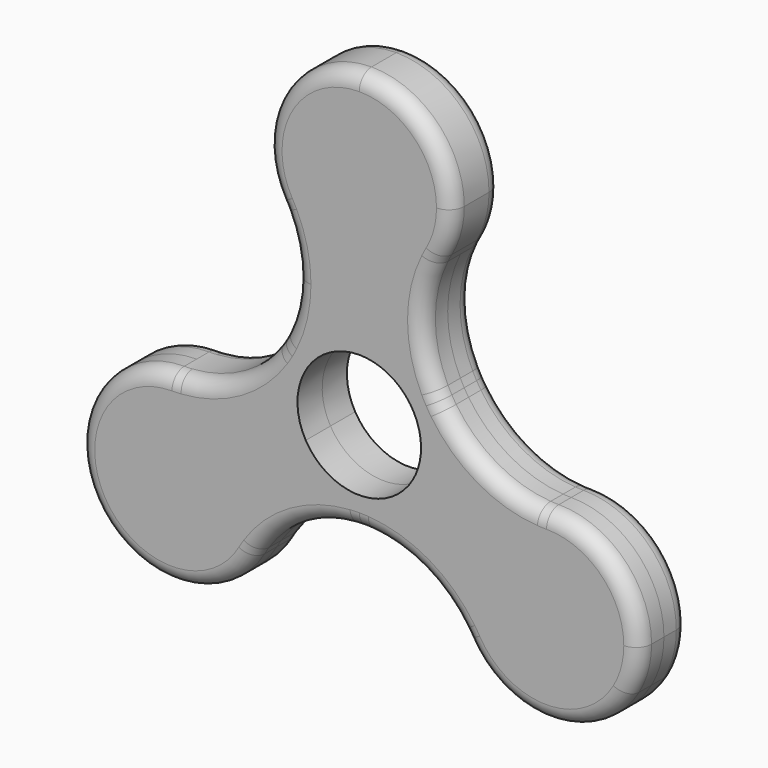
from build123d import *

# Parameters (mm, degrees)
F1_DEPTH = 2.54
F2_R     = 1.27


# Not quite as in the source:
# - a feature names something its author has since deleted; it is built from what else it names


with BuildPart() as f1:
    # F0 (on Front) → F1 (new body, symmetric)
    with BuildSketch(Plane.XZ):
        with BuildLine():
            ThreePointArc((7.62, 17.78), (5.3881536726, 23.1681536726), (0, 25.4))
            Line((0, 25.4), (0, 10.16))
            ThreePointArc((0, 10.16), (3.249178877, 10.887450644), (5.877985768, 12.9309090222))
            ThreePointArc((5.877985768, 12.9309090222), (6.260146038, 13.4354664712), (6.5991134209, 13.96999973))
            ThreePointArc((6.5991134209, 13.96999973), (7.360354756, 15.8077987257), (7.62, 17.78))
        make_face()
        with BuildLine():
            Line((0, 10.16), (0, 25.4))
            ThreePointArc((0, 25.4), (-6.5991135286, 21.5900000836), (-6.5991136733, 13.9700001671))
            ThreePointArc((-6.5991136733, 13.9700001671), (-6.2601461875, 13.4354666866), (-5.8779857805, 12.9309090373))
            ThreePointArc((-5.8779857805, 12.9309090373), (-3.2491788858, 10.8874506481), (0, 10.16))
        make_face()
        with BuildLine():
            Line((0, 7.62), (0, 10.16))
            ThreePointArc((0, 10.16), (-3.2491788858, 10.8874506481), (-5.8779857805, 12.9309090373))
            ThreePointArc((-5.8779857805, 12.9309090373), (-4.8002366489, 11.0368765758), (-4.4263073453, 8.89))
            ThreePointArc((-4.4263073453, 8.89), (-4.8002366648, 6.74312338), (-5.8779858402, 4.8490908903))
            ThreePointArc((-5.8779858402, 4.8490908903), (-3.2491789283, 6.8925493318), (0, 7.62))
        make_face()
        with BuildLine():
            ThreePointArc((5.877985768, 12.9309090222), (3.249178877, 10.887450644), (0, 10.16))
            Line((0, 10.16), (0, 7.62))
            ThreePointArc((0, 7.62), (3.2491789453, 6.8925493238), (5.8779858642, 4.8490908613))
            ThreePointArc((5.8779858642, 4.8490908613), (4.4263073453, 8.8899999245), (5.877985768, 12.9309090222))
        make_face()
        with BuildLine():
            ThreePointArc((-14.1374887376, -1.3749694884), (-11.0533983396, -2.6298538308), (-8.7988181024, -5.08))
            Line((-8.7988181024, -5.08), (-6.5991135768, -3.81))
            ThreePointArc((-6.5991135768, -3.81), (-7.5937122775, -0.6324032306), (-7.1384288571, 2.6659395065))
            ThreePointArc((-7.1384288571, 2.6659395065), (-9.9121195778, -0.6117054319), (-14.1374887376, -1.3749694884))
        make_face()
        with BuildLine():
            Line((-6.5991135768, -3.81), (-8.7988181024, -5.08))
            ThreePointArc((-8.7988181024, -5.08), (-8.037576883, -6.9177988763), (-7.7779316793, -8.89))
            ThreePointArc((-7.7779316793, -8.89), (-7.8992908924, -10.2445428561), (-8.2595028995, -11.5559397134))
            ThreePointArc((-8.2595028995, -11.5559397134), (-5.4858122449, -8.2782946509), (-1.2604430504, -7.5150304934))
            ThreePointArc((-1.2604430504, -7.5150304934), (-4.344533385, -6.2601461378), (-6.5991135768, -3.81))
        make_face()
        with BuildLine():
            ThreePointArc((-15.3979316793, -1.27), (-21.9970452561, -5.08), (-21.9970452561, -12.7))
            Line((-21.9970452561, -12.7), (-8.7988181024, -5.08))
            ThreePointArc((-8.7988181024, -5.08), (-11.0533983396, -2.6298538308), (-14.1374887376, -1.3749694884))
            ThreePointArc((-14.1374887376, -1.3749694884), (-14.7655285241, -1.2962877162), (-15.3979316793, -1.27))
        make_face()
        with BuildLine():
            Line((-8.7988181024, -5.08), (-21.9970452561, -12.7))
            ThreePointArc((-21.9970452561, -12.7), (-15.3979316818, -16.51), (-8.7988181049, -12.7000000043))
            ThreePointArc((-8.7988181049, -12.7000000043), (-8.5053823708, -12.1391789778), (-8.2595028995, -11.5559397134))
            ThreePointArc((-8.2595028995, -11.5559397134), (-7.8992908924, -10.2445428561), (-7.7779316793, -8.89))
            ThreePointArc((-7.7779316793, -8.89), (-8.037576883, -6.9177988763), (-8.7988181024, -5.08))
        make_face()
        with BuildLine():
            ThreePointArc((1.2604429732, -7.5150305063), (4.3445333529, -6.2601461601), (6.5991135768, -3.81))
            Line((6.5991135768, -3.81), (4.3994090512, -2.54))
            ThreePointArc((4.3994090512, -2.54), (0, -5.08), (-4.3994090512, -2.54))
            Line((-4.3994090512, -2.54), (-6.5991135768, -3.81))
            ThreePointArc((-6.5991135768, -3.81), (-4.344533385, -6.2601461378), (-1.2604430504, -7.5150304934))
            ThreePointArc((-1.2604430504, -7.5150304934), (-0.6324032184, -7.5937122785), (-1.66e-08, -7.62))
            ThreePointArc((-1.66e-08, -7.62), (0.6324031628, -7.5937122832), (1.2604429732, -7.5150305063))
        make_face()
        with BuildLine():
            Line((-6.5991135768, -3.81), (-4.3994090512, -2.54))
            ThreePointArc((-4.3994090512, -2.54), (-4.3994090512, 2.54), (0, 5.08))
            Line((0, 5.08), (0, 7.62))
            ThreePointArc((0, 7.62), (-3.2491789283, 6.8925493318), (-5.8779858402, 4.8490908903))
            ThreePointArc((-5.8779858402, 4.8490908903), (-6.2601461212, 4.3445334089), (-6.5991135101, 3.8100001156))
            ThreePointArc((-6.5991135101, 3.8100001156), (-6.8925493282, 3.249178936), (-7.1384288571, 2.6659395065))
            ThreePointArc((-7.1384288571, 2.6659395065), (-7.5937122775, -0.6324032306), (-6.5991135768, -3.81))
        make_face()
        with BuildLine():
            ThreePointArc((8.2595029011, -11.5559397177), (7.8042193924, -8.2575968818), (8.7988181024, -5.08))
            Line((8.7988181024, -5.08), (6.5991135768, -3.81))
            ThreePointArc((6.5991135768, -3.81), (4.3445333529, -6.2601461601), (1.2604429732, -7.5150305063))
            ThreePointArc((1.2604429732, -7.5150305063), (5.4858122129, -8.2782946325), (8.2595029011, -11.5559397177))
        make_face()
        with BuildLine():
            Line((6.5991135768, -3.81), (8.7988181024, -5.08))
            ThreePointArc((8.7988181024, -5.08), (11.0533983038, -2.6298538556), (14.1374886517, -1.3749695028))
            ThreePointArc((14.1374886517, -1.3749695028), (9.9121195513, -0.6117054166), (7.1384288662, 2.6659394822))
            ThreePointArc((7.1384288662, 2.6659394822), (7.4986408088, 1.3545427346), (7.62, 0))
            ThreePointArc((7.62, 0), (7.3603547963, -1.9722011237), (6.5991135768, -3.81))
        make_face()
        with BuildLine():
            Line((8.7988181024, -5.08), (21.9970452561, -12.7))
            ThreePointArc((21.9970452561, -12.7), (22.7582864756, -10.8622011237), (23.0179316793, -8.89))
            ThreePointArc((23.0179316793, -8.89), (20.7860853519, -3.5018463274), (15.3979316793, -1.27))
            ThreePointArc((15.3979316793, -1.27), (14.7655284807, -1.2962877198), (14.1374886517, -1.3749695028))
            ThreePointArc((14.1374886517, -1.3749695028), (11.0533983038, -2.6298538556), (8.7988181024, -5.08))
        make_face()
        with BuildLine():
            ThreePointArc((8.7988181117, -12.700000016), (15.3979316885, -16.51), (21.9970452561, -12.7))
            Line((21.9970452561, -12.7), (8.7988181024, -5.08))
            ThreePointArc((8.7988181024, -5.08), (7.8042193924, -8.2575968818), (8.2595029011, -11.5559397177))
            ThreePointArc((8.2595029011, -11.5559397177), (8.5053823746, -12.139178986), (8.7988181117, -12.700000016))
        make_face()
        with BuildLine():
            ThreePointArc((-14.7246582835, -1.2476675293), (-14.4325799527, -1.318266846), (-14.1374887376, -1.3749694884))
            ThreePointArc((-14.1374887376, -1.3749694884), (-9.9121195778, -0.6117054319), (-7.1384288571, 2.6659395065))
            ThreePointArc((-7.1384288571, 2.6659395065), (-7.0399891484, 2.9498473861), (-6.9550907617, 3.2380943709))
            ThreePointArc((-6.9550907617, 3.2380943709), (-10.3179316793, 0.0911818976), (-14.7246582835, -1.2476675293))
        make_face()
        with BuildLine():
            Line((4.3994090512, -2.54), (6.5991135768, -3.81))
            ThreePointArc((6.5991135768, -3.81), (7.3603547963, -1.9722011237), (7.62, 0))
            ThreePointArc((7.62, 0), (7.4986408088, 1.3545427346), (7.1384288662, 2.6659394822))
            ThreePointArc((7.1384288662, 2.6659394822), (6.8925492974, 3.2491790013), (6.5991134249, 3.8100002632))
            ThreePointArc((6.5991134249, 3.8100002632), (6.2601460834, 4.3445334634), (5.8779858642, 4.8490908613))
            ThreePointArc((5.8779858642, 4.8490908613), (3.2491789453, 6.8925493238), (0, 7.62))
            Line((0, 7.62), (0, 5.08))
            ThreePointArc((0, 5.08), (3.5921024484, 3.5921024484), (5.08, 0))
            ThreePointArc((5.08, 0), (4.9069031975, -1.3148007491), (4.3994090512, -2.54))
        make_face()
        with BuildLine():
            ThreePointArc((-1.2604430504, -7.5150304934), (-5.4858122449, -8.2782946509), (-8.2595028995, -11.5559397134))
            ThreePointArc((-8.2595028995, -11.5559397134), (-8.3579425646, -11.8398474913), (-8.4428409176, -12.1280943709))
            ThreePointArc((-8.4428409176, -12.1280943709), (-5.08, -8.9811818976), (-0.6732733958, -7.6423324707))
            ThreePointArc((-0.6732733958, -7.6423324707), (-0.9653517805, -7.5717331423), (-1.2604430504, -7.5150304934))
        make_face()
        with BuildLine():
            ThreePointArc((8.4428409176, -12.1280943709), (8.3579425653, -11.8398474934), (8.2595029011, -11.5559397177))
            ThreePointArc((8.2595029011, -11.5559397177), (5.4858122129, -8.2782946325), (1.2604429732, -7.5150305063))
            ThreePointArc((1.2604429732, -7.5150305063), (0.9653517422, -7.5717331506), (0.6732733958, -7.6423324707))
            ThreePointArc((0.6732733958, -7.6423324707), (5.08, -8.9811818976), (8.4428409176, -12.1280943709))
        make_face()
        with BuildLine():
            ThreePointArc((7.1384288662, 2.6659394822), (9.9121195513, -0.6117054166), (14.1374886517, -1.3749695028))
            ThreePointArc((14.1374886517, -1.3749695028), (14.4325799101, -1.3182668553), (14.7246582835, -1.2476675293))
            ThreePointArc((14.7246582835, -1.2476675293), (10.3179316793, 0.0911818976), (6.9550907617, 3.2380943709))
            ThreePointArc((6.9550907617, 3.2380943709), (7.0399891524, 2.9498473737), (7.1384288662, 2.6659394822))
        make_face()
        with BuildLine():
            ThreePointArc((6.2818173659, 13.3757619002), (6.0746373488, 13.1581142492), (5.877985768, 12.9309090222))
            ThreePointArc((5.877985768, 12.9309090222), (4.4263073453, 8.8899999245), (5.8779858642, 4.8490908613))
            ThreePointArc((5.8779858642, 4.8490908613), (6.0746373996, 4.6218856948), (6.2818173659, 4.4042380998))
            ThreePointArc((6.2818173659, 4.4042380998), (5.2379316793, 8.89), (6.2818173659, 13.3757619002))
        make_face()
        with BuildLine():
            ThreePointArc((-4.4263073453, 8.89), (-4.8002366489, 11.0368765758), (-5.8779857805, 12.9309090373))
            ThreePointArc((-5.8779857805, 12.9309090373), (-6.0746373554, 13.1581142565), (-6.2818173659, 13.3757619002))
            ThreePointArc((-6.2818173659, 13.3757619002), (-5.5023437376, 11.1928111707), (-5.2379316793, 8.89))
            ThreePointArc((-5.2379316793, 8.89), (-5.5023437376, 6.5871888293), (-6.2818173659, 4.4042380998))
            ThreePointArc((-6.2818173659, 4.4042380998), (-6.074637387, 4.6218857087), (-5.8779858402, 4.8490908903))
            ThreePointArc((-5.8779858402, 4.8490908903), (-4.8002366648, 6.74312338), (-4.4263073453, 8.89))
        make_face()
        with BuildLine():
            ThreePointArc((-8.2595028995, -11.5559397134), (-8.5053823708, -12.1391789778), (-8.7988181049, -12.7000000043))
            ThreePointArc((-8.7988181049, -12.7000000043), (-8.6255707333, -12.4110960593), (-8.4428409176, -12.1280943709))
            ThreePointArc((-8.4428409176, -12.1280943709), (-8.3579425646, -11.8398474913), (-8.2595028995, -11.5559397134))
        make_face()
        with BuildLine():
            ThreePointArc((-0.6732733958, -7.6423324707), (-0.3368218472, -7.6255846528), (-1.66e-08, -7.62))
            ThreePointArc((-1.66e-08, -7.62), (-0.6324032184, -7.5937122785), (-1.2604430504, -7.5150304934))
            ThreePointArc((-1.2604430504, -7.5150304934), (-0.9653517805, -7.5717331423), (-0.6732733958, -7.6423324707))
        make_face()
        with BuildLine():
            ThreePointArc((0.6732733958, -7.6423324707), (0.9653517422, -7.5717331506), (1.2604429732, -7.5150305063))
            ThreePointArc((1.2604429732, -7.5150305063), (0.6324031628, -7.5937122832), (-1.66e-08, -7.62))
            ThreePointArc((-1.66e-08, -7.62), (0.3368218306, -7.6255846523), (0.6732733958, -7.6423324707))
        make_face()
        with BuildLine():
            ThreePointArc((-14.7246582835, -1.2476675293), (-15.0611098403, -1.2644153475), (-15.3979316793, -1.27))
            ThreePointArc((-15.3979316793, -1.27), (-14.7655285241, -1.2962877162), (-14.1374887376, -1.3749694884))
            ThreePointArc((-14.1374887376, -1.3749694884), (-14.4325799527, -1.318266846), (-14.7246582835, -1.2476675293))
        make_face()
        with BuildLine():
            ThreePointArc((-6.9550907617, 3.2380943709), (-7.0399891484, 2.9498473861), (-7.1384288571, 2.6659395065))
            ThreePointArc((-7.1384288571, 2.6659395065), (-6.8925493282, 3.249178936), (-6.5991135101, 3.8100001156))
            ThreePointArc((-6.5991135101, 3.8100001156), (-6.772360912, 3.5210961139), (-6.9550907617, 3.2380943709))
        make_face()
        with BuildLine():
            ThreePointArc((-6.5991135101, 3.8100001156), (-6.2601461212, 4.3445334089), (-5.8779858402, 4.8490908903))
            ThreePointArc((-5.8779858402, 4.8490908903), (-6.074637387, 4.6218857087), (-6.2818173659, 4.4042380998))
            ThreePointArc((-6.2818173659, 4.4042380998), (-6.4355390769, 4.1044886542), (-6.5991135101, 3.8100001156))
        make_face()
        with BuildLine():
            ThreePointArc((-5.8779857805, 12.9309090373), (-6.2601461875, 13.4354666866), (-6.5991136733, 13.9700001671))
            ThreePointArc((-6.5991136733, 13.9700001671), (-6.4355391538, 13.6755114898), (-6.2818173659, 13.3757619002))
            ThreePointArc((-6.2818173659, 13.3757619002), (-6.0746373554, 13.1581142565), (-5.8779857805, 12.9309090373))
        make_face()
        with BuildLine():
            ThreePointArc((6.2818173659, 13.3757619002), (6.4355390349, 13.6755112671), (6.5991134209, 13.96999973))
            ThreePointArc((6.5991134209, 13.96999973), (6.260146038, 13.4354664712), (5.877985768, 12.9309090222))
            ThreePointArc((5.877985768, 12.9309090222), (6.0746373488, 13.1581142492), (6.2818173659, 13.3757619002))
        make_face()
        with BuildLine():
            ThreePointArc((5.8779858642, 4.8490908613), (6.2601460834, 4.3445334634), (6.5991134249, 3.8100002632))
            ThreePointArc((6.5991134249, 3.8100002632), (6.4355390368, 4.1044887294), (6.2818173659, 4.4042380998))
            ThreePointArc((6.2818173659, 4.4042380998), (6.0746373996, 4.6218856948), (5.8779858642, 4.8490908613))
        make_face()
        with BuildLine():
            ThreePointArc((6.5991134249, 3.8100002632), (6.8925492974, 3.2491790013), (7.1384288662, 2.6659394822))
            ThreePointArc((7.1384288662, 2.6659394822), (7.0399891524, 2.9498473737), (6.9550907617, 3.2380943709))
            ThreePointArc((6.9550907617, 3.2380943709), (6.772360867, 3.5210961862), (6.5991134249, 3.8100002632))
        make_face()
        with BuildLine():
            ThreePointArc((14.7246582835, -1.2476675293), (14.4325799101, -1.3182668553), (14.1374886517, -1.3749695028))
            ThreePointArc((14.1374886517, -1.3749695028), (14.7655284807, -1.2962877198), (15.3979316793, -1.27))
            ThreePointArc((15.3979316793, -1.27), (15.0611098403, -1.2644153475), (14.7246582835, -1.2476675293))
        make_face()
        with BuildLine():
            ThreePointArc((8.4428409176, -12.1280943709), (8.6255707369, -12.411096065), (8.7988181117, -12.700000016))
            ThreePointArc((8.7988181117, -12.700000016), (8.5053823746, -12.139178986), (8.2595029011, -11.5559397177))
            ThreePointArc((8.2595029011, -11.5559397177), (8.3579425653, -11.8398474934), (8.4428409176, -12.1280943709))
        make_face()
    extrude(amount=F1_DEPTH, both=True)

    # F2
    f2_edges = [f1.edges().sort_by_distance(p)[0] for p in [
        (0, 2.54, -7.62),
        (6.599114, -2.54, 3.81),
    ]]
    fillet(f2_edges, radius=F2_R)


solid = f1.part
